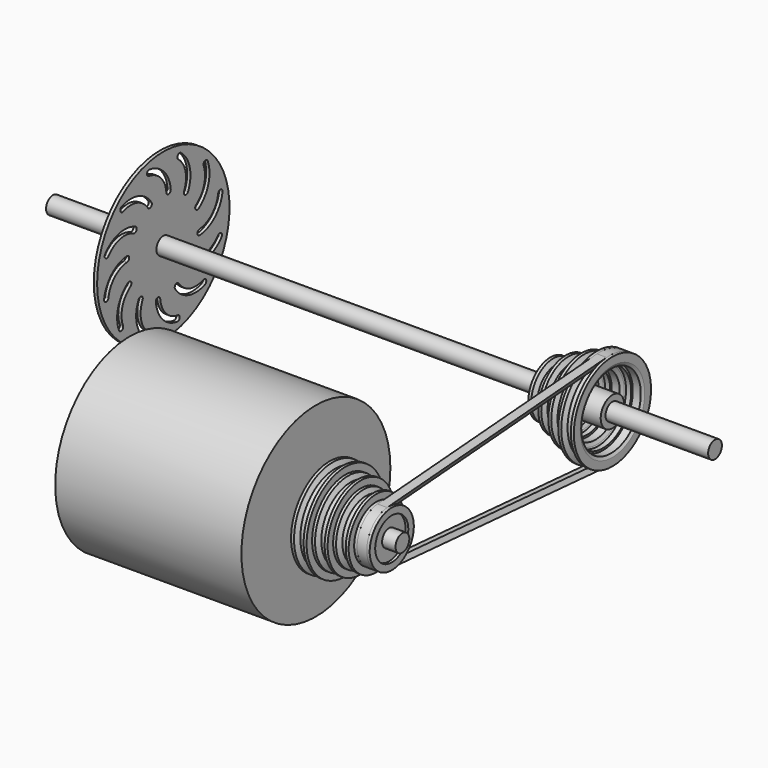
from build123d import *

# Parameters (mm, degrees)
F1_W           = 184.15
F1_H           = 7.9375
F1_W_2         = 3.175
F9_T           = 5.588
F7_R           = 7.9375
F10_DEPTH      = 508
F10_DEPTH_BACK = 101.6
F12_R          = 76.2
F13_DEPTH      = 3.048


# Not quite as in the source:
# - a shell that OpenCascade refuses in one call is made with other operations: the cavity is built on its own and cut out


with BuildPart() as f2:
    # F1 (on Top) → F2 (revolve)
    with BuildSketch(Plane.XY):
        Polygon((-92.075, 25.4), (-92.075, 7.9375), (92.075, 7.9375), (92.075, 25.4), (85.725, 25.4), (85.725, 85.725), (-85.725, 85.725), (-85.725, 25.4), align=None)
    revolve(axis=Axis((127.7326234779, 0, 0), (1, 0, 0)))


with BuildPart() as f3:
    # F1 (on Top) → F3 (revolve)
    with BuildSketch(Plane.XY):
        Polygon((92.075, 7.9375), (92.075, 0), (165.3904053223, 0), (165.3904053223, 7.9375), (153.035, 7.9375), (98.425, 7.9375), align=None)
        with Locations((0, 3.96875)):
            Rectangle(F1_W, F1_H)
        with Locations((-93.6625, 3.96875)):
            Rectangle(F1_W_2, F1_H)
    revolve(axis=Axis((127.7326234779, 0, 0), (1, 0, 0)))


with BuildPart() as f4:
    # F1 (on Top) → F4 (revolve)
    with BuildSketch(Plane.XY):
        Polygon((98.425, 44.45), (98.425, 7.9375), (153.035, 7.9375), (153.035, 19.05), (155.575, 19.05), (155.575, 25.4), (152.87625, 25.4), (150.71725, 20.828), (146.14525, 20.828), (143.98625, 25.4), (141.2875, 25.4), (141.2875, 31.75), (138.58875, 31.75), (136.42975, 27.178), (131.85775, 27.178), (129.69875, 31.75), (127, 31.75), (127, 38.1), (124.30125, 38.1), (122.14225, 33.528), (117.57025, 33.528), (115.41125, 38.1), (112.7125, 38.1), (112.7125, 44.45), (110.01375, 44.45), (107.85475, 39.878), (103.28275, 39.878), (101.12375, 44.45), align=None)
    revolve(axis=Axis((127.7326234779, 0, 0), (1, 0, 0)))


with BuildPart() as f5:
    # F1 (on Top) → F5 (revolve)
    with BuildSketch(Plane.XY):
        Polygon((103.28275, 233.172), (107.85475, 233.172), (110.01375, 228.6), (112.7125, 228.6), (112.7125, 222.25), (115.41125, 222.25), (117.57025, 226.822), (122.14225, 226.822), (124.30125, 222.25), (127, 222.25), (127, 215.9), (129.69875, 215.9), (131.85775, 220.472), (136.42975, 220.472), (138.58875, 215.9), (141.2875, 215.9), (141.2875, 209.55), (143.98625, 209.55), (146.14525, 214.122), (150.71725, 214.122), (152.87625, 209.55), (155.575, 209.55), (155.575, 246.0625), (100.965, 246.0625), (100.965, 234.95), (98.425, 234.95), (98.425, 228.6), (101.12375, 228.6), align=None)
    revolve(axis=Axis((126.2673765221, 254, 0), (-1, 0, 0)))

    # F9: shell of thickness 5.588, made by hand


with BuildPart() as f8:
    # F8: sweep along a path in F7
    with BuildLine(Plane.YZ.offset(148.43125)) as f8_path:
        Line((250.66625, 44.3248080756), (-1.905, 25.3284617575))
        ThreePointArc((-1.905, 25.3284617575), (-25.4, 0), (-1.905, -25.3284617575))
        Line((-1.905, -25.3284617575), (250.66625, -44.3248080756))
        ThreePointArc((250.66625, -44.3248080756), (298.45, 0), (250.66625, 44.3248080756))
    # F1 (on Top) → F8 (sweep)
    with BuildSketch(Plane.XY):
        Polygon((152.87625, -25.4), (150.71725, -20.828), (146.14525, -20.828), (143.98625, -25.4), align=None)
    sweep(path=f8_path.line)


with BuildPart() as f9_core1:
    # F9_t2: copy of F5
    add(f5.part)

    # the walls: a layer under each face that stays
    f9_faces = [f9_core1.faces().sort_by_distance(p)[0] for p in [
        (105.56875, 274.828, 0),
        (108.93425, 277.114, 0),
        (111.363125, 279.4, 0),
        (112.7125, 232.8333333333, -21.1666666667),
        (114.061875, 285.75, 0),
        (116.49075, 283.464, 0),
        (119.85625, 281.178, 0),
        (123.22175, 283.464, 0),
        (125.650625, 285.75, 0),
        (127, 228.6, -25.4),
        (128.349375, 292.1, 0),
        (130.77825, 289.814, 0),
        (134.14375, 287.528, 0),
        (137.50925, 289.814, 0),
        (139.938125, 292.1, 0),
        (141.2875, 224.3666666667, -29.6333333333),
        (142.636875, 298.45, 0),
        (145.06575, 296.164, 0),
        (148.43125, 293.878, 0),
        (151.79675, 296.164, 0),
        (154.225625, 298.45, 0),
        (128.27, 261.9375, 0),
        (100.965, 241.3, -12.7),
        (99.695, 273.05, 0),
        (98.425, 237.0666666667, -16.9333333333),
        (99.774375, 279.4, 0),
        (102.20325, 277.114, 0),
    ]]
    thicken(f9_faces, amount=-F9_T, mode=Mode.SUBTRACT)

    # F9_s3 → F9_t4 (revolve, cut)
    with BuildSketch(Plane.XY):
        Polygon((103.3332794144, 233.0922588877), (103.28275, 238.76), (99.7418115901, 238.76), (98.229808562, 235.5581112346), align=None)
    revolve(axis=Axis((103.28275, 254, 0), (-1, 0, 0)), mode=Mode.SUBTRACT)

    # F9_s5 → F9_t6 (revolve, cut)
    with BuildSketch(Plane.XY):
        Polygon((107.8042205856, 233.0922588877), (107.85475, 238.76), (111.3956884099, 238.76), (112.907691438, 235.5581112346), align=None)
    revolve(axis=Axis((107.85475, 254, 0), (-1, 0, 0)), mode=Mode.SUBTRACT)

    # F9_s7 → F9_t8 (revolve, cut)
    with BuildSketch(Plane.XY):
        Polygon((112.65662, 228.54412), (112.7125, 234.188), (118.3005, 234.188), (118.3005, 228.6), align=None)
    revolve(axis=Axis((112.7125, 254, 0), (-1, 0, 0)), mode=Mode.SUBTRACT)

    # F9_s9 → F9_t10 (revolve, cut)
    with BuildSketch(Plane.XY):
        Polygon((117.6207794144, 226.7422588877), (112.517308562, 229.2081112346), (114.0293115901, 232.41), (117.57025, 232.41), align=None)
    revolve(axis=Axis((117.57025, 254, 0), (-1, 0, 0)), mode=Mode.SUBTRACT)

    # F9_s11 → F9_t12 (revolve, cut)
    with BuildSketch(Plane.XY):
        Polygon((122.0917205856, 226.7422588877), (122.14225, 232.41), (125.6831884099, 232.41), (127.195191438, 229.2081112346), align=None)
    revolve(axis=Axis((122.14225, 254, 0), (-1, 0, 0)), mode=Mode.SUBTRACT)

    # F9_s13 → F9_t14 (revolve, cut)
    with BuildSketch(Plane.XY):
        Polygon((126.94412, 222.19412), (127, 227.838), (132.588, 227.838), (132.588, 222.25), align=None)
    revolve(axis=Axis((127, 254, 0), (-1, 0, 0)), mode=Mode.SUBTRACT)

    # F9_s15 → F9_t16 (revolve, cut)
    with BuildSketch(Plane.XY):
        Polygon((131.9082794144, 220.3922588877), (126.804808562, 222.8581112346), (128.3168115901, 226.06), (131.85775, 226.06), align=None)
    revolve(axis=Axis((131.85775, 254, 0), (-1, 0, 0)), mode=Mode.SUBTRACT)

    # F9_s17 → F9_t18 (revolve, cut)
    with BuildSketch(Plane.XY):
        Polygon((136.3792205856, 220.3922588877), (136.42975, 226.06), (139.9706884099, 226.06), (141.482691438, 222.8581112346), align=None)
    revolve(axis=Axis((136.42975, 254, 0), (-1, 0, 0)), mode=Mode.SUBTRACT)

    # F9_s19 → F9_t20 (revolve, cut)
    with BuildSketch(Plane.XY):
        Polygon((141.23162, 215.84412), (141.2875, 221.488), (146.8755, 221.488), (146.8755, 215.9), align=None)
    revolve(axis=Axis((141.2875, 254, 0), (-1, 0, 0)), mode=Mode.SUBTRACT)

    # F9_s21 → F9_t22 (revolve, cut)
    with BuildSketch(Plane.XY):
        Polygon((146.1957794144, 214.0422588877), (141.092308562, 216.5081112346), (142.6043115901, 219.71), (146.14525, 219.71), align=None)
    revolve(axis=Axis((146.14525, 254, 0), (-1, 0, 0)), mode=Mode.SUBTRACT)

    # F9_s23 → F9_t24 (revolve, cut)
    with BuildSketch(Plane.XY):
        Polygon((150.6667205856, 214.0422588877), (150.71725, 219.71), (154.2581884099, 219.71), (155.770191438, 216.5081112346), align=None)
    revolve(axis=Axis((150.71725, 254, 0), (-1, 0, 0)), mode=Mode.SUBTRACT)

    # F9_s25 → F9_t26 (revolve, cut)
    with BuildSketch(Plane.XY):
        Polygon((100.90912, 235.00588), (106.553, 234.95), (106.553, 229.362), (100.965, 229.362), align=None)
    revolve(axis=Axis((100.965, 254, 0), (-1, 0, 0)), mode=Mode.SUBTRACT)


with BuildPart() as f5_1:
    add(f5.part)

    # what is left inside the walls is the cavity
    f9_cavity = [f9_core1.part.solids().sort_by_distance(p)[0] for p in [
        (139.234333, 267.58138, 0),
    ]]
    add(f9_cavity, mode=Mode.SUBTRACT)


with BuildPart() as f10:
    # F7 (on plane+point) → F10 (new body, two sides)
    with BuildSketch(Plane.YZ.offset(148.43125)) as f10_sk:
        with Locations((254, 0)):
            Circle(F7_R)
    extrude(amount=-F10_DEPTH)
    extrude(f10_sk.sketch, amount=F10_DEPTH_BACK)


with BuildPart() as f13:
    # F12 (on offset) → F13 (new body)
    with BuildSketch(Plane(origin=(-257.96875, 0, 0), x_dir=(0, -1, 0), z_dir=(-1, 0, 0))):
        with Locations((-254, 0)):
            Circle(F12_R)
        with BuildLine():
            ThreePointArc((-267.5626688922, -40.6626399469), (-282.8856706329, -51.9278104434), (-301.8854255326, -51.0865242797))
            ThreePointArc((-301.8854255326, -51.0865242797), (-303.2910319935, -47.78085181), (-299.9853595238, -46.3752453491))
            ThreePointArc((-299.9853595238, -46.3752453491), (-284.3618975797, -47.0670333449), (-271.7618226931, -37.8037052928))
            ThreePointArc((-271.7618226931, -37.8037052928), (-268.2327784656, -37.1335957194), (-267.5626688922, -40.6626399469))
        make_face(mode=Mode.SUBTRACT)
        with BuildLine():
            ThreePointArc((-245.4142958303, -41.9962136251), (-253.0518193517, -59.4136383233), (-269.9267328424, -68.1849405836))
            ThreePointArc((-269.9267328424, -68.1849405836), (-272.7968599801, -66.0249474786), (-270.6368668752, -63.1548203409))
            ThreePointArc((-270.6368668752, -63.1548203409), (-256.7606579387, -55.9421953473), (-250.4803370233, -41.6198804873))
            ThreePointArc((-250.4803370233, -41.6198804873), (-247.7591498579, -39.2750264597), (-245.4142958303, -41.9962136251))
        make_face(mode=Mode.SUBTRACT)
        with BuildLine():
            ThreePointArc((-286.0769357772, -28.4335447329), (-304.9796297951, -30.5279676904), (-321.0132571221, -20.2995150509))
            ThreePointArc((-321.0132571221, -20.2995150509), (-320.5777117901, -16.7339154851), (-317.0121122243, -17.1694608171))
            ThreePointArc((-317.0121122243, -17.1694608171), (-303.8276912836, -25.5802977676), (-288.2840423161, -23.8580577942))
            ThreePointArc((-288.2840423161, -23.8580577942), (-284.8927455773, -25.0422479941), (-286.0769357772, -28.4335447329))
        make_face(mode=Mode.SUBTRACT)
        with BuildLine():
            ThreePointArc((-225.5664552671, -32.0769357772), (-223.4720323096, -50.9796297951), (-233.7004849491, -67.0132571221))
            ThreePointArc((-233.7004849491, -67.0132571221), (-237.2660845149, -66.5777117901), (-236.8305391829, -63.0121122243))
            ThreePointArc((-236.8305391829, -63.0121122243), (-228.4197022324, -49.8276912836), (-230.1419422058, -34.2840423161))
            ThreePointArc((-230.1419422058, -34.2840423161), (-228.9577520059, -30.8927455773), (-225.5664552671, -32.0769357772))
        make_face(mode=Mode.SUBTRACT)
        with BuildLine():
            ThreePointArc((-213.3373600531, -13.5626688922), (-202.0721895566, -28.8856706329), (-202.9134757203, -47.8854255326))
            ThreePointArc((-202.9134757203, -47.8854255326), (-206.21914819, -49.2910319935), (-207.6247546509, -45.9853595238))
            ThreePointArc((-207.6247546509, -45.9853595238), (-206.9329666551, -30.3618975797), (-216.1962947072, -17.7618226931))
            ThreePointArc((-216.1962947072, -17.7618226931), (-216.8664042806, -14.2327784656), (-213.3373600531, -13.5626688922))
        make_face(mode=Mode.SUBTRACT)
        with BuildLine():
            ThreePointArc((-212.0037863749, 8.5857041697), (-194.5863616767, 0.9481806483), (-185.8150594164, -15.9267328424))
            ThreePointArc((-185.8150594164, -15.9267328424), (-187.9750525214, -18.7968599801), (-190.8451796591, -16.6368668752))
            ThreePointArc((-190.8451796591, -16.6368668752), (-198.0578046527, -2.7606579387), (-212.3801195127, 3.5196629767))
            ThreePointArc((-212.3801195127, 3.5196629767), (-214.7249735403, 6.2408501421), (-212.0037863749, 8.5857041697))
        make_face(mode=Mode.SUBTRACT)
        with BuildLine():
            ThreePointArc((-317.1548203409, 16.6368668752), (-309.9421953473, 2.7606579387), (-295.6198804873, -3.5196629767))
            ThreePointArc((-295.6198804873, -3.5196629767), (-293.2750264597, -6.2408501421), (-295.9962136251, -8.5857041697))
            ThreePointArc((-295.9962136251, -8.5857041697), (-313.4136383233, -0.9481806483), (-322.1849405836, 15.9267328424))
            ThreePointArc((-322.1849405836, 15.9267328424), (-320.0249474786, 18.7968599801), (-317.1548203409, 16.6368668752))
        make_face(mode=Mode.SUBTRACT)
        with BuildLine():
            ThreePointArc((-294.6626399469, 13.5626688922), (-305.9278104434, 28.8856706329), (-305.0865242797, 47.8854255326))
            ThreePointArc((-305.0865242797, 47.8854255326), (-301.78085181, 49.2910319935), (-300.3752453491, 45.9853595238))
            ThreePointArc((-300.3752453491, 45.9853595238), (-301.0670333449, 30.3618975797), (-291.8037052928, 17.7618226931))
            ThreePointArc((-291.8037052928, 17.7618226931), (-291.1335957194, 14.2327784656), (-294.6626399469, 13.5626688922))
        make_face(mode=Mode.SUBTRACT)
        with BuildLine():
            ThreePointArc((-282.4335447329, 32.0769357772), (-284.5279676904, 50.9796297951), (-274.2995150509, 67.0132571221))
            ThreePointArc((-274.2995150509, 67.0132571221), (-270.7339154851, 66.5777117901), (-271.1694608171, 63.0121122243))
            ThreePointArc((-271.1694608171, 63.0121122243), (-279.5802977676, 49.8276912836), (-277.8580577942, 34.2840423161))
            ThreePointArc((-277.8580577942, 34.2840423161), (-279.0422479941, 30.8927455773), (-282.4335447329, 32.0769357772))
        make_face(mode=Mode.SUBTRACT)
        with BuildLine():
            ThreePointArc((-221.9230642228, 28.4335447329), (-203.0203702049, 30.5279676904), (-186.9867428779, 20.2995150509))
            ThreePointArc((-186.9867428779, 20.2995150509), (-187.4222882099, 16.7339154851), (-190.9878877757, 17.1694608171))
            ThreePointArc((-190.9878877757, 17.1694608171), (-204.1723087164, 25.5802977676), (-219.7159576839, 23.8580577942))
            ThreePointArc((-219.7159576839, 23.8580577942), (-223.1072544227, 25.0422479941), (-221.9230642228, 28.4335447329))
        make_face(mode=Mode.SUBTRACT)
        with BuildLine():
            ThreePointArc((-262.5857041697, 41.9962136251), (-254.9481806483, 59.4136383233), (-238.0732671576, 68.1849405836))
            ThreePointArc((-238.0732671576, 68.1849405836), (-235.2031400199, 66.0249474786), (-237.3631331248, 63.1548203409))
            ThreePointArc((-237.3631331248, 63.1548203409), (-251.2393420613, 55.9421953473), (-257.5196629767, 41.6198804873))
            ThreePointArc((-257.5196629767, 41.6198804873), (-260.2408501421, 39.2750264597), (-262.5857041697, 41.9962136251))
        make_face(mode=Mode.SUBTRACT)
        with BuildLine():
            ThreePointArc((-240.4373311078, 40.6626399469), (-225.1143293671, 51.9278104434), (-206.1145744674, 51.0865242797))
            ThreePointArc((-206.1145744674, 51.0865242797), (-204.7089680065, 47.78085181), (-208.0146404762, 46.3752453491))
            ThreePointArc((-208.0146404762, 46.3752453491), (-223.6381024203, 47.0670333449), (-236.2381773069, 37.8037052928))
            ThreePointArc((-236.2381773069, 37.8037052928), (-239.7672215344, 37.1335957194), (-240.4373311078, 40.6626399469))
        make_face(mode=Mode.SUBTRACT)
    extrude(amount=F13_DEPTH)


solid = Compound([f2.part, f3.part, f4.part, f8.part, f5_1.part, f10.part, f13.part])
